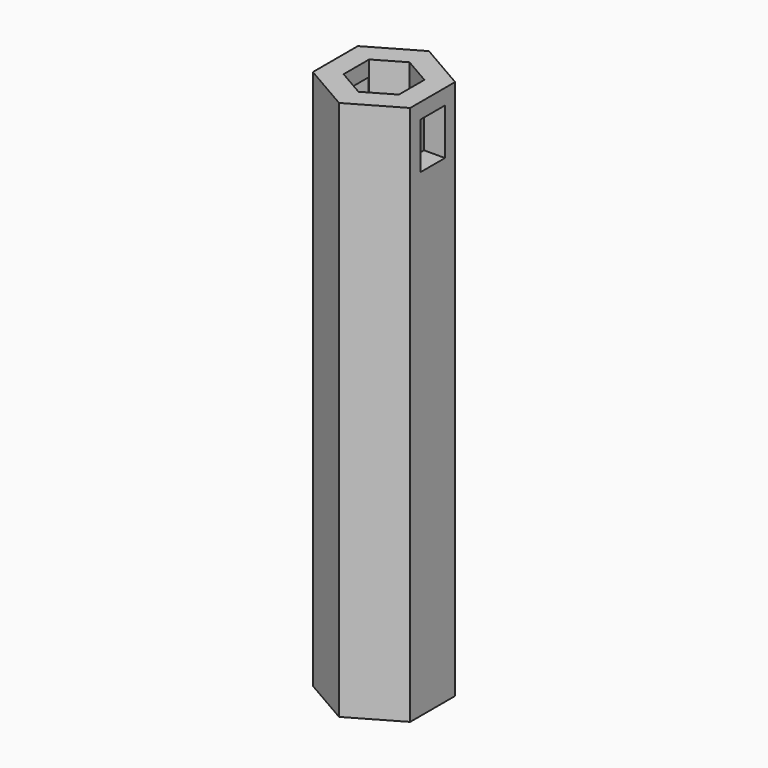
from build123d import *

# Parameters (mm, degrees)
F1_DEPTH      = 25
F1_DEPTH_BACK = 10
F3_DEPTH      = 25
F5_DEPTH      = 13.6
F5_DEPTH_BACK = 25


with BuildPart() as f1:
    # F0 (on Top) → F1 (new body, two sides)
    with BuildSketch(Plane.XY) as f1_sk:
        Polygon((-3.15, 1.8186533479), (-3.15, -1.8186533479), (0, -3.6373066959), (3.15, -1.8186533479), (3.15, 1.8186533479), (0, 3.6373066959), align=None)
    extrude(amount=F1_DEPTH)
    extrude(f1_sk.sketch, amount=-F1_DEPTH_BACK)

    # F2 (on Top) → F3 (cut)
    with BuildSketch(Plane.XY):
        Polygon((-1.79, 1.0334569818), (-1.79, -1.0334569818), (0, -2.0669139637), (1.79, -1.0334569818), (1.79, 1.0334569818), (0, 2.0669139637), align=None)
    extrude(amount=F3_DEPTH, mode=Mode.SUBTRACT)

    # F4 (on Right) → F5 (cut, two sides)
    with BuildSketch(Plane.YZ) as f5_sk:
        Polygon((-1, 21), (0, 21), (1, 21), (1, 24), (0, 24), (-1, 24), align=None)
    extrude(amount=-F5_DEPTH, mode=Mode.SUBTRACT)
    extrude(f5_sk.sketch, amount=F5_DEPTH_BACK, mode=Mode.SUBTRACT)


solid = f1.part
